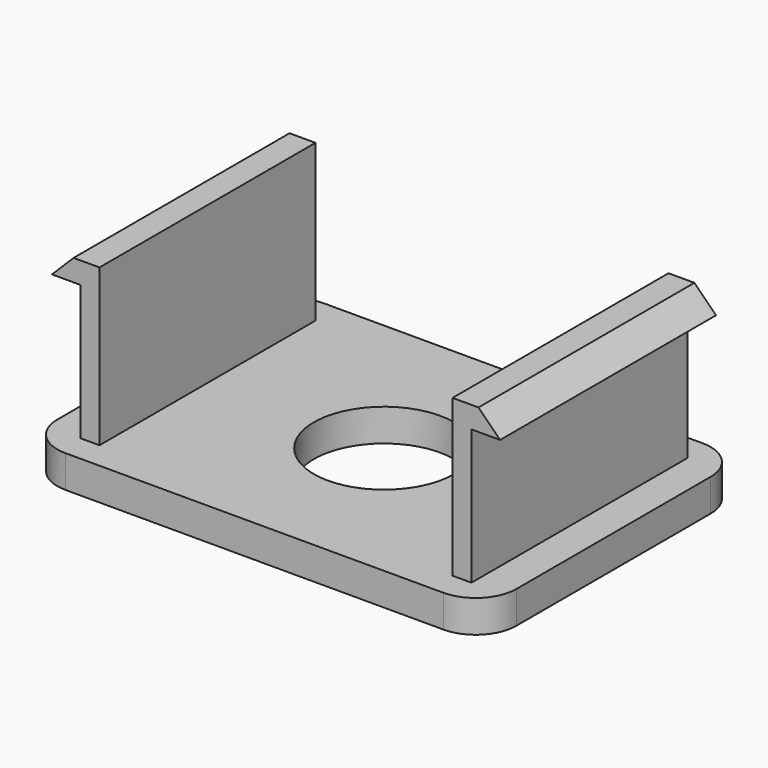
from build123d import *

# Parameters (mm, degrees)
F0_W        = 21.59
F0_H        = 15.24
F0_W_2      = 0.889
F0_H_2      = 12.7
F0_R        = 3.302
F1_DEPTH    = 1.524
F2_DEPTH    = 8.89
F3_W        = 12.7
F3_H        = 1.016
F5_DEPTH    = 1.6002
F4_W        = 12.7
F4_H        = 1.016
F6_DEPTH    = 1.6002
F7_T1_DEPTH = 19.2320747894
F8_R        = 1.905


# Not quite as in the source:
# - a fillet or chamfer that OpenCascade refuses, or shapes differently, is made with other operations: its cross-section is extruded or revolved along the edge and cut away or added


with BuildPart() as f1:
    # F0 (on Top) → F1 (new body)
    with BuildSketch(Plane.XY):
        Rectangle(F0_W, F0_H)
        with Locations((-8.7503, 0)):
            Rectangle(F0_W_2, F0_H_2, mode=Mode.SUBTRACT)
        Circle(F0_R, mode=Mode.SUBTRACT)
        with Locations((8.7503, 0)):
            Rectangle(F0_W_2, F0_H_2, mode=Mode.SUBTRACT)
    extrude(amount=F1_DEPTH)

    # F0 (on Top) → F2 (join)
    with BuildSketch(Plane.XY):
        with Locations((-8.7503, 0)):
            Rectangle(F0_W_2, F0_H_2)
        with Locations((8.7503, 0)):
            Rectangle(F0_W_2, F0_H_2)
    extrude(amount=F2_DEPTH)

    # F3 (on face) → F5 (join)
    with BuildSketch(Plane(origin=(-9.1948, 0, 0), x_dir=(0, -1, 0), z_dir=(-1, 0, 0))):
        with Locations((0, 8.382)):
            Rectangle(F3_W, F3_H)
    extrude(amount=F5_DEPTH)

    # F4 (on face) → F6 (join)
    with BuildSketch(Plane.YZ.offset(9.1948)):
        with Locations((0, 8.382)):
            Rectangle(F4_W, F4_H)
    extrude(amount=F6_DEPTH)

    # F7: chamfer of 1.27 on 2 edges, made by hand

    # F7_s2 → F7_t1 (cut)
    with BuildSketch(Plane.XZ.offset(-9.6160373947)):
        Polygon((-10.795, 7.62), (-9.525, 8.89), (-10.795, 8.89), align=None)
        Polygon((10.795, 7.62), (9.525, 8.89), (10.795, 8.89), align=None)
    extrude(amount=F7_T1_DEPTH, mode=Mode.SUBTRACT)

    # F8
    f8_edges = [f1.edges().sort_by_distance(p)[0] for p in [
        (10.795, -7.62, 0.762),
        (10.795, 7.62, 0.762),
        (-10.795, 7.62, 0.762),
        (-10.795, -7.62, 0.762),
    ]]
    fillet(f8_edges, radius=F8_R)


solid = f1.part
